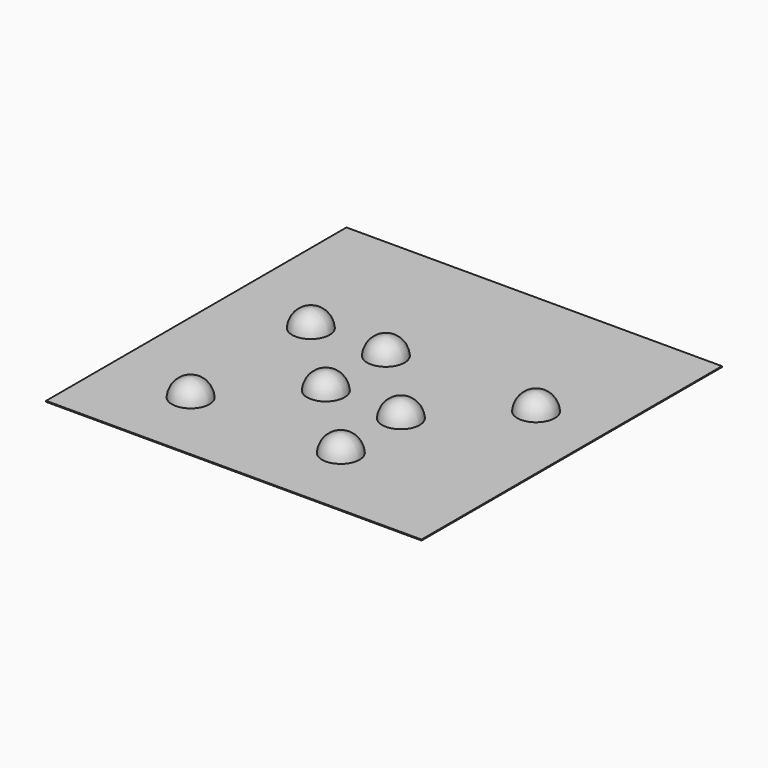
from build123d import *

# Parameters (mm, degrees)
F1_W     = 200
F1_H     = 200
F1_R     = 10
F2_DEPTH = 0.5
F3_DEPTH = 10


# Not quite as in the source:
# - a fillet or chamfer that OpenCascade refuses, or shapes differently, is made with other operations: its cross-section is extruded or revolved along the edge and cut away or added


with BuildPart() as f2:
    # F1 (on face) → F2 (new body)
    with BuildSketch(Plane.XY):
        Rectangle(F1_W, F1_H)
        with Locations((-55, -60)):
            Circle(F1_R, mode=Mode.SUBTRACT)
        with Locations((-15, -20)):
            Circle(F1_R, mode=Mode.SUBTRACT)
        with Locations((25, -60)):
            Circle(F1_R, mode=Mode.SUBTRACT)
        with Locations((25, -20)):
            Circle(F1_R, mode=Mode.SUBTRACT)
        with Locations((-55, 20)):
            Circle(F1_R, mode=Mode.SUBTRACT)
        with Locations((-15, 20)):
            Circle(F1_R, mode=Mode.SUBTRACT)
        with Locations((65, 20)):
            Circle(F1_R, mode=Mode.SUBTRACT)
    extrude(amount=F2_DEPTH)

    # F1 (on face) → F3 (join)
    with BuildSketch(Plane.XY):
        with Locations((-55, -60)):
            Circle(F1_R)
        with Locations((-55, 20)):
            Circle(F1_R)
        with Locations((-15, -20)):
            Circle(F1_R)
        with Locations((-15, 20)):
            Circle(F1_R)
        with Locations((25, -60)):
            Circle(F1_R)
        with Locations((25, -20)):
            Circle(F1_R)
        with Locations((65, 20)):
            Circle(F1_R)
    extrude(amount=F3_DEPTH)

    # F4: fillet of radius 10 on 7 edges, made by hand

    # F4_s1 → F4_t2 (revolve, cut)
    with BuildSketch(Plane.XZ.offset(-20)):
        with BuildLine():
            ThreePointArc((-45, 0.5), (-48.0954678017, 7.2456883731), (-54.9874921777, 10))
            Line((-54.9874921777, 10), (-45, 10))
            Line((-45, 10), (-45, 0.5))
        make_face()
    revolve(axis=Axis((-55, 20, 10), (0, 0, 1)), mode=Mode.SUBTRACT)

    # F4_s3 → F4_t4 (revolve, cut)
    with BuildSketch(Plane.XZ.offset(-20)):
        with BuildLine():
            ThreePointArc((-5, 0.5), (-8.0954678017, 7.2456883731), (-14.9874921777, 10))
            Line((-14.9874921777, 10), (-5, 10))
            Line((-5, 10), (-5, 0.5))
        make_face()
    revolve(axis=Axis((-15, 20, 10), (0, 0, 1)), mode=Mode.SUBTRACT)

    # F4_s5 → F4_t6 (revolve, cut)
    with BuildSketch(Plane.XZ.offset(-20)):
        with BuildLine():
            ThreePointArc((75, 0.5), (71.9045321983, 7.2456883731), (65.0125078223, 10))
            Line((65.0125078223, 10), (75, 10))
            Line((75, 10), (75, 0.5))
        make_face()
    revolve(axis=Axis((65, 20, 10), (0, 0, 1)), mode=Mode.SUBTRACT)

    # F4_s7 → F4_t8 (revolve, cut)
    with BuildSketch(Plane.XZ.offset(20)):
        with BuildLine():
            ThreePointArc((35, 0.5), (31.9045321983, 7.2456883731), (25.0125078223, 10))
            Line((25.0125078223, 10), (35, 10))
            Line((35, 10), (35, 0.5))
        make_face()
    revolve(axis=Axis((25, -20, 10), (0, 0, 1)), mode=Mode.SUBTRACT)

    # F4_s9 → F4_t10 (revolve, cut)
    with BuildSketch(Plane.XZ.offset(20)):
        with BuildLine():
            ThreePointArc((-5, 0.5), (-8.0954678017, 7.2456883731), (-14.9874921777, 10))
            Line((-14.9874921777, 10), (-5, 10))
            Line((-5, 10), (-5, 0.5))
        make_face()
    revolve(axis=Axis((-15, -20, 10), (0, 0, 1)), mode=Mode.SUBTRACT)

    # F4_s11 → F4_t12 (revolve, cut)
    with BuildSketch(Plane.XZ.offset(60)):
        with BuildLine():
            ThreePointArc((-45, 0.5), (-48.0954678017, 7.2456883731), (-54.9874921777, 10))
            Line((-54.9874921777, 10), (-45, 10))
            Line((-45, 10), (-45, 0.5))
        make_face()
    revolve(axis=Axis((-55, -60, 10), (0, 0, 1)), mode=Mode.SUBTRACT)

    # F4_s13 → F4_t14 (revolve, cut)
    with BuildSketch(Plane.XZ.offset(60)):
        with BuildLine():
            ThreePointArc((35, 0.5), (31.9045321983, 7.2456883731), (25.0125078223, 10))
            Line((25.0125078223, 10), (35, 10))
            Line((35, 10), (35, 0.5))
        make_face()
    revolve(axis=Axis((25, -60, 10), (0, 0, 1)), mode=Mode.SUBTRACT)


solid = f2.part
